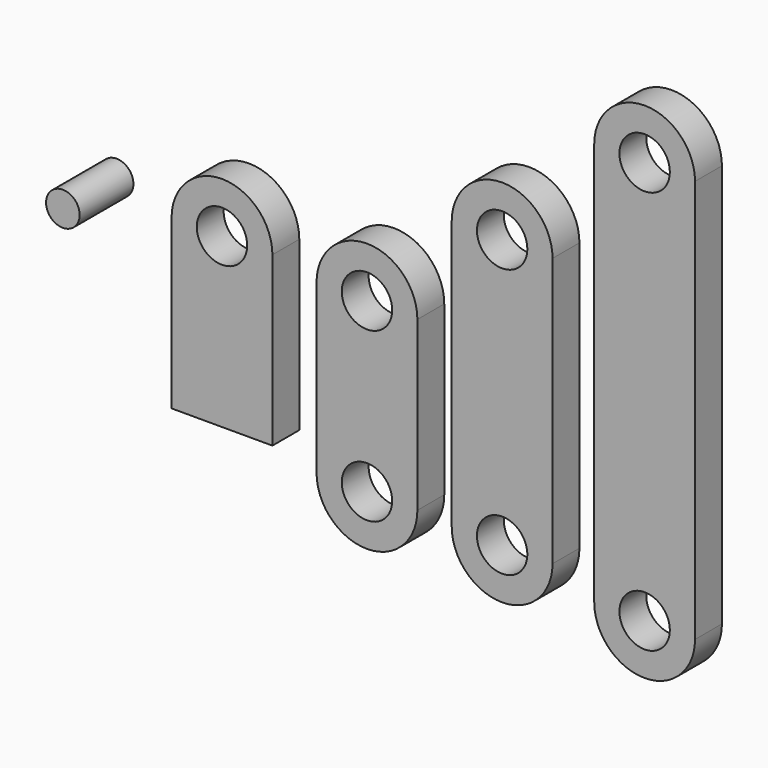
from build123d import *

# Parameters (mm, degrees)
F1_R      = 190.5
F2_DEPTH  = 254
F3_R      = 190.5
F4_DEPTH  = 254
F5_R      = 190.5
F6_DEPTH  = 254
F7_R      = 190.5
F8_DEPTH  = 254
F9_R      = 127
F10_DEPTH = 508


# Not quite as in the source:
# - a variable given as a bare number and used for a length is read in inches; the dataset says mm whatever the document's units were


with BuildPart() as f2:
    # F1 (on Front) → F2 (new body)
    with BuildSketch(Plane.XZ):
        with BuildLine():
            Line((350.0158497542, -1230.4982659221), (350.0158497542, 39.5017340779))
            ThreePointArc((350.0158497542, 39.5017340779), (-30.9841502458, 420.5017340779), (-411.9841502458, 39.5017340779))
            Line((-411.9841502458, 39.5017340779), (-411.9841502458, -1230.4982659221))
            Line((-411.9841502458, -1230.4982659221), (350.0158497542, -1230.4982659221))
        make_face()
        with Locations((-30.9841502458, 39.5017340779)):
            Circle(F1_R, mode=Mode.SUBTRACT)
    extrude(amount=F2_DEPTH)


with BuildPart() as f4:
    # F3 (on Front) → F4 (new body)
    with BuildSketch(Plane.XZ):
        with BuildLine():
            Line((1445.8497519493, -1304.3150901794), (1445.8497519493, -34.3150901794))
            ThreePointArc((1445.8497519493, -34.3150901794), (1064.8497519493, 346.6849098206), (683.8497519493, -34.3150901794))
            Line((683.8497519493, -34.3150901794), (683.8497519493, -1304.3150901794))
            ThreePointArc((683.8497519493, -1304.3150901794), (1064.8497519493, -1685.3150901794), (1445.8497519493, -1304.3150901794))
        make_face()
        with Locations((1064.8497519493, -1304.3150901794)):
            Circle(F3_R, mode=Mode.SUBTRACT)
        with Locations((1064.8497519493, -34.3150901794)):
            Circle(F3_R, mode=Mode.SUBTRACT)
    extrude(amount=F4_DEPTH)


with BuildPart() as f6:
    # F5 (on Front) → F6 (new body)
    with BuildSketch(Plane.XZ):
        with BuildLine():
            Line((2467.521941185, -1327.6220560074), (2467.521941185, 704.3779439926))
            ThreePointArc((2467.521941185, 704.3779439926), (2086.521941185, 1085.3779439926), (1705.521941185, 704.3779439926))
            Line((1705.521941185, 704.3779439926), (1705.521941185, -1327.6220560074))
            ThreePointArc((1705.521941185, -1327.6220560074), (2086.521941185, -1708.6220560074), (2467.521941185, -1327.6220560074))
        make_face()
        with Locations((2086.521941185, -1327.6220560074)):
            Circle(F5_R, mode=Mode.SUBTRACT)
        with Locations((2086.521941185, 704.3779439926)):
            Circle(F5_R, mode=Mode.SUBTRACT)
    extrude(amount=F6_DEPTH)


with BuildPart() as f8:
    # F7 (on Front) → F8 (new body)
    with BuildSketch(Plane.XZ):
        with BuildLine():
            Line((3544.5384140015, -1480.9713363647), (3544.5384140015, 1567.0286636353))
            ThreePointArc((3544.5384140015, 1567.0286636353), (3163.5384140015, 1948.0286636353), (2782.5384140015, 1567.0286636353))
            Line((2782.5384140015, 1567.0286636353), (2782.5384140015, -1480.9713363647))
            ThreePointArc((2782.5384140015, -1480.9713363647), (3163.5384140015, -1861.9713363647), (3544.5384140015, -1480.9713363647))
        make_face()
        with Locations((3163.5384140015, -1480.9713363647)):
            Circle(F7_R, mode=Mode.SUBTRACT)
        with Locations((3163.5384140015, 1567.0286636353)):
            Circle(F7_R, mode=Mode.SUBTRACT)
    extrude(amount=F8_DEPTH)


with BuildPart() as f10:
    # F9 (on Front) → F10 (new body)
    with BuildSketch(Plane.XZ):
        with Locations((-1030.6034088135, 0)):
            Circle(F9_R)
    extrude(amount=F10_DEPTH)


solid = Compound([f2.part, f4.part, f6.part, f8.part, f10.part])
